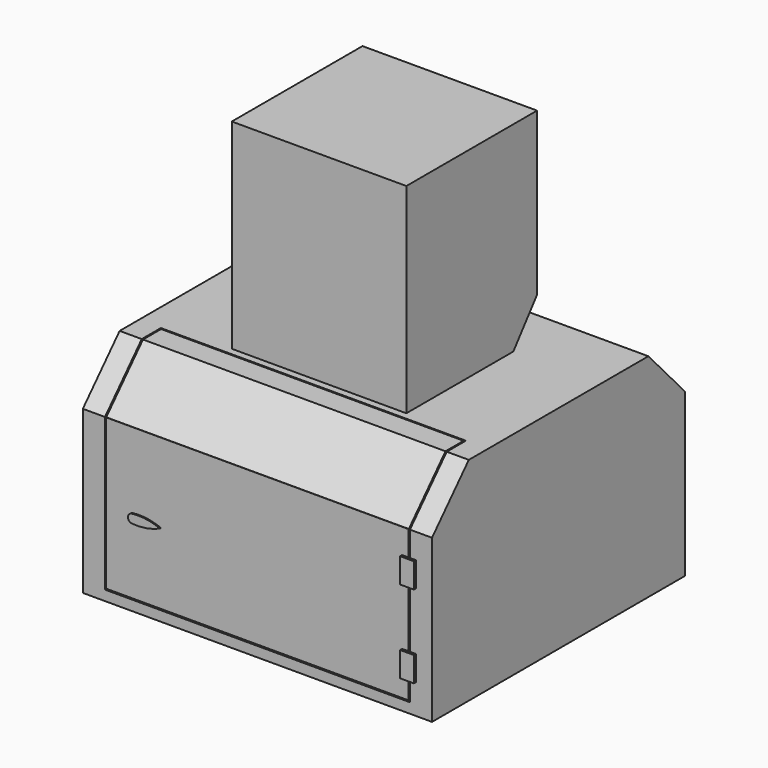
from build123d import *

# Parameters (mm, degrees)
F0_W      = 700
F0_H      = 650
F0_W_2    = 670
F0_H_2    = 620
F1_DEPTH  = 650
F3_DEPTH  = 700
F4_W      = 1400
F4_H      = 900
F4_W_2    = 700
F4_H_2    = 531.2062842084
F5_DEPTH  = 200
F7_DEPTH  = 1400
F8_W      = 1399.7949943277
F8_H      = 1268.6949958977
F8_W_2    = 700
F8_H_2    = 531.2062842084
F9_DEPTH  = 650
F10_W     = 1222.8473691637
F10_H     = 0.4061281681
F10_W_2   = 1212.8473691637
F10_H_2   = 5
F11_DEPTH = 25
F12_W     = 5
F12_H     = 271.4476656914
F13_DEPTH = 25
F15_DEPTH = 25
F16_R     = 11.3345027625
F17_DEPTH = 5
F18_DEPTH = 10
F20_DEPTH = 5
F21_W     = 668
F21_H     = 499.1960943538
F22_DEPTH = 170
F23_W     = 700
F23_H     = 802.1854579449
F24_DEPTH = 5
F26_DEPTH = 1175
F28_DEPTH = 250
F30_DEPTH = 250


# Not quite as in the source:
# - a feature names something its author has since deleted; it is built from what else it names


with BuildPart() as f1:
    # F0 (on Front) → F1 (new body)
    with BuildSketch(Plane.XZ):
        Rectangle(F0_W, F0_H)
        Rectangle(F0_W_2, F0_H_2, mode=Mode.SUBTRACT)
    extrude(amount=-F1_DEPTH)

    # F2 (on face) → F3 (join)
    with BuildSketch(Plane.YZ.offset(350)):
        Polygon((531.2062842084, -477.1854579449), (650, -325), (0, -325), (0, -477.1854579449), align=None)
    extrude(amount=-F3_DEPTH)

    # F21 (on face) → F22 (cut)
    with BuildSketch(Plane(origin=(0, 0, -477.1854579449), x_dir=(1, 0, 0), z_dir=(0, 0, -1))):
        with Locations((0, -265.7305951914)):
            Rectangle(F21_W, F21_H)
    extrude(amount=-F22_DEPTH, mode=Mode.SUBTRACT)

    # F23 (on face) → F24 (join)
    with BuildSketch(Plane.XZ):
        with Locations((0, -76.0927289724)):
            Rectangle(F23_W, F23_H)
    extrude(amount=F24_DEPTH)


with BuildPart() as f5:
    # F4 (on face) → F5 (new body)
    with BuildSketch(Plane(origin=(0, 0, -477.1854579449), x_dir=(1, 0, 0), z_dir=(0, 0, -1))):
        with Locations((0, -320.3603625298)):
            Rectangle(F4_W, F4_H)
        with Locations((0, -265.6031421042)):
            Rectangle(F4_W_2, F4_H_2, mode=Mode.SUBTRACT)
    extrude(amount=F5_DEPTH)

    # F6 (on face) → F7 (join)
    with BuildSketch(Plane.YZ.offset(700)):
        Polygon((-129.6396374702, -677.1854579449), (-129.6396374702, -477.1854579449), (-313.9871354191, -677.1854579449), align=None)
        Polygon((770.3603625298, -477.1854579449), (770.3603625298, -677.1854579449), (954.7078604786, -677.1854579449), align=None)
    extrude(amount=-F7_DEPTH)

    # F8 (on face) → F9 (join)
    with BuildSketch(Plane(origin=(0, 0, -677.1854579449), x_dir=(1, 0, 0), z_dir=(0, 0, -1))):
        with Locations((0.1025028361, -320.3603625298)):
            Rectangle(F8_W, F8_H)
        with Locations((0, -265.6031421042)):
            Rectangle(F8_W_2, F8_H_2, mode=Mode.SUBTRACT)
    extrude(amount=F9_DEPTH)

    # F10 (on face) → F11 (cut)
    with BuildSketch(Plane.XZ.offset(313.9871354191)):
        with Locations((0.1025028361, -1327.3885220289)):
            Rectangle(F10_W, F10_H)
        Polygon((-606.3211817457, -677.1854579449), (-611.3211817457, -677.1854579449), (-611.3211817457, -1286.6218090057), (-606.3211817457, -1286.6218090057), (-606.3211817457, -1281.6218090057), align=None)
        Polygon((611.526187418, -1286.6218090057), (611.526187418, -677.1854579449), (606.526187418, -677.1854579449), (606.526187418, -1281.6218090057), (606.526187418, -1286.6218090057), align=None)
        Polygon((611.526187418, -676.7793297768), (-611.3211817457, -676.7793297768), (-611.3211817457, -677.1854579449), (-606.3211817457, -677.1854579449), (606.526187418, -677.1854579449), (611.526187418, -677.1854579449), align=None)
        with Locations((0.1025028361, -1284.1218090057)):
            Rectangle(F10_W_2, F10_H_2)
    extrude(amount=-F11_DEPTH, mode=Mode.SUBTRACT)

    # F12 (on face) → F13 (cut)
    with BuildSketch(Plane(origin=(0, 167.7119856609, -154.5864246631), x_dir=(1, 0, 0), z_dir=(0, -0.7352941176, 0.6777481542))):
        with Locations((609.026187418, -574.458518109)):
            Rectangle(F12_W, F12_H)
        with Locations((-608.8211817457, -574.458518109)):
            Rectangle(F12_W, F12_H)
    extrude(amount=-F13_DEPTH, mode=Mode.SUBTRACT)

    # F14 (on face) → F15 (cut)
    with BuildSketch(Plane.XY.offset(-477.1854579449)):
        Polygon((611.526187418, -33.8904465006), (-611.3211817457, -33.8904465006), (-611.3211817457, -129.6396374702), (-606.3211817457, -129.6396374702), (-606.3211817457, -38.8904465006), (606.526187418, -38.8904465006), (606.526187418, -129.6396374702), (611.526187418, -129.6396374702), align=None)
    extrude(amount=-F15_DEPTH, mode=Mode.SUBTRACT)

    # F16 (on face) → F17 (join)
    with BuildSketch(Plane.XZ.offset(313.9871354191)):
        Polygon((635, -1108.2031965256), (580, -1108.2031965256), (580, -1208.2031965256), (635, -1208.2031965256), (635, -1168.8231229782), align=None)
        Polygon((635, -777.1854579449), (580, -777.1854579449), (580, -877.1854579449), (635, -877.1854579449), (635, -808.090031147), align=None)
        with Locations((-489.5007610321, -990.9374713898)):
            Circle(F16_R)
    extrude(amount=F17_DEPTH)

    # F16 (on face) → F18 (join)
    with BuildSketch(Plane.XZ.offset(313.9871354191)):
        Polygon((635, -1108.2031965256), (580, -1108.2031965256), (580, -1208.2031965256), (635, -1208.2031965256), (635, -1168.8231229782), align=None)
        Polygon((635, -777.1854579449), (580, -777.1854579449), (580, -877.1854579449), (635, -877.1854579449), (635, -808.090031147), align=None)
        with Locations((-489.5007610321, -990.9374713898)):
            Circle(F16_R)
    extrude(amount=F18_DEPTH)

    # F19 (on face) → F20 (join)
    with BuildSketch(Plane.XZ.offset(323.9871354191)):
        with BuildLine():
            ThreePointArc((-489.5007610321, -1008.5250073511), (-477.0644950895, -1003.3737373324), (-471.9132250707, -990.9374713898))
            ThreePointArc((-471.9132250707, -990.9374713898), (-477.5624320948, -978.0224520952), (-490.8809444539, -973.4041740697))
            ThreePointArc((-490.8809444539, -973.4041740697), (-507.074732102, -991.6280957645), (-489.5007610321, -1008.5250073511))
        make_face()
        with BuildLine():
            ThreePointArc((-490.8809444539, -973.4041740697), (-477.5624320948, -978.0224520952), (-471.9132250707, -990.9374713898))
            ThreePointArc((-471.9132250707, -990.9374713898), (-477.0644950895, -1003.3737373324), (-489.5007610321, -1008.5250073511))
            ThreePointArc((-489.5007610321, -1008.5250073511), (-432.8396587778, -1005.9231706341), (-378.5828948021, -989.3867373466))
            ThreePointArc((-378.5828948021, -989.3867373466), (-433.7199381181, -974.2849848856), (-490.8809444539, -973.4041740697))
        make_face()
    extrude(amount=F20_DEPTH)

    # F25 (on face) → F26 (join)
    with BuildSketch(Plane.YZ.offset(700)):
        Polygon((173.9625222218, -1373.4135972352), (0, -1327.1854579449), (-9.543454825, -1327.1854579449), (183.7482365325, -1378.5500571563), align=None)
        Polygon((541.05185, -1327.1854579449), (530, -1327.1854579449), (311.4313689114, -1378.5500571563), (322.4832189114, -1378.5500571563), align=None)
    extrude(amount=-F26_DEPTH)

    # F27 (on face) → F28 (cut)
    with BuildSketch(Plane.YZ.offset(700)):
        Polygon((-9.543454825, -1327.1854579449), (183.7482365325, -1378.5500571563), (173.9625222218, -1373.4135972352), (0, -1327.1854579449), align=None)
    extrude(amount=-F28_DEPTH, mode=Mode.SUBTRACT)

    # F29 (on face) → F30 (cut)
    with BuildSketch(Plane.YZ.offset(700)):
        Polygon((530, -1327.1854579449), (311.4313689114, -1378.5500571563), (322.4832189114, -1378.5500571563), (541.05185, -1327.1854579449), align=None)
    extrude(amount=-F30_DEPTH, mode=Mode.SUBTRACT)


solid = Compound([f1.part, f5.part])
